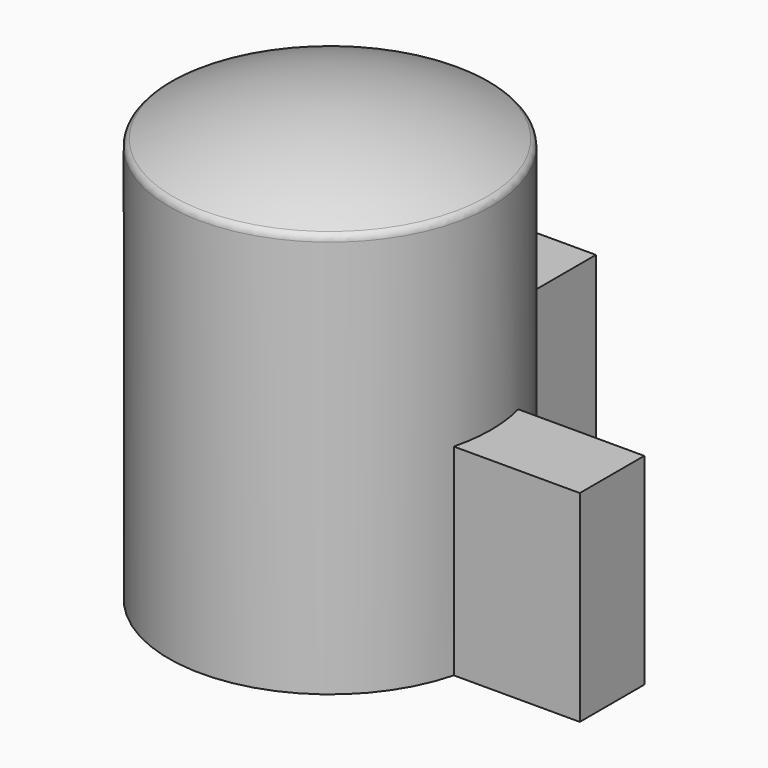
from build123d import *

# Parameters (mm, degrees)
F2_R     = 0.2
F4_DEPTH = 5


with BuildPart() as f1:
    # F0 (on Front) → F1 (revolve)
    with BuildSketch(Plane.XZ):
        with BuildLine():
            Line((0, 9.25), (0, 0))
            Line((0, 0), (4, 0))
            Line((4, 0), (4, 10))
            Line((4, 10), (3.75, 10))
            ThreePointArc((3.75, 10), (1.9121323176, 9.439338412), (0, 9.25))
        make_face()
        with BuildLine():
            Line((0, 10), (0, 9.25))
            ThreePointArc((0, 9.25), (1.9121323176, 9.439338412), (3.75, 10))
            Line((3.75, 10), (0, 10))
        make_face()
        with BuildLine():
            Line((3.75, 10), (4, 10))
            ThreePointArc((4, 10), (2.0615528128, 10.7462112512), (0, 11))
            Line((0, 11), (0, 10))
            Line((0, 10), (3.75, 10))
        make_face()
    revolve(axis=Axis((0, 0, 5), (0, 0, -1)))

    # F2
    f2_edges = [f1.edges().sort_by_distance(p)[0] for p in [
        (-4, 0, 10),
    ]]
    fillet(f2_edges, radius=F2_R)

    # F3 (on Top) → F4 (join)
    with BuildSketch(Plane.XY):
        Polygon((-1, 7), (-1, 0), (0, 0), (0, 1), (1, 1), (1, 7), align=None)
        Polygon((1, 0), (0, 0), (0, -1), (7, -1), (7, 1), (1, 1), align=None)
    extrude(amount=F4_DEPTH)


solid = f1.part
